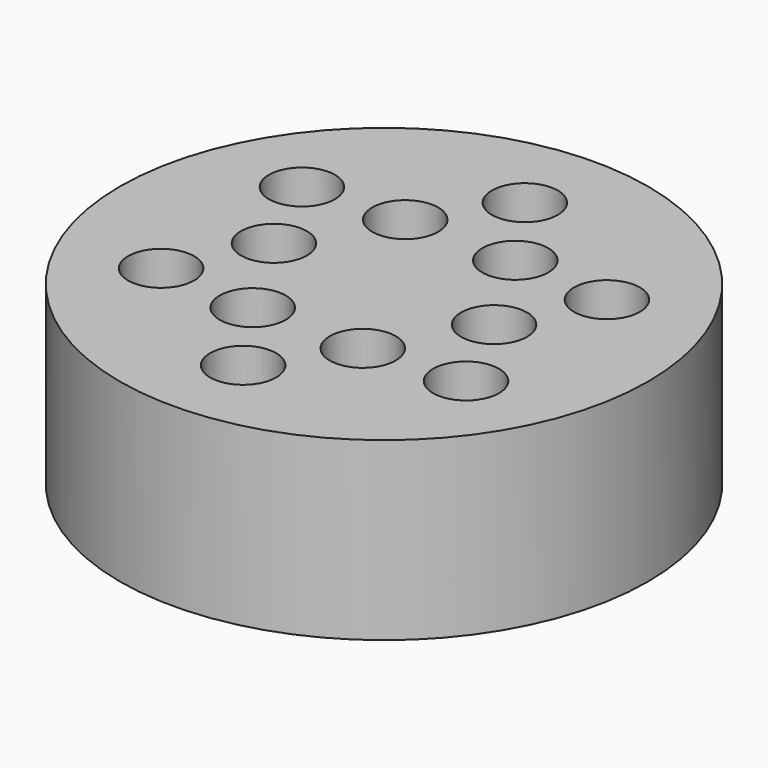
from build123d import *

# Parameters (mm, degrees)
F0_R     = 60
F1_DEPTH = 40
F2_R     = 7.5
F3_DEPTH = 25
F4_R     = 7.5
F5_DEPTH = 40.001


# Not quite as in the source:
# - a feature names something its author has since deleted; it is built from what else it names


with BuildPart() as f1:
    # F0 (on Top) → F1 (new body)
    with BuildSketch(Plane.XY):
        Circle(F0_R)
    extrude(amount=F1_DEPTH)

    # F2 (on face) → F3 (cut)
    with BuildSketch(Plane.XY.offset(40)):
        with Locations((-34.6410161514, 20)):
            Circle(F2_R)
        with Locations((0, 40)):
            Circle(F2_R)
        with Locations((34.6410161514, 20)):
            Circle(F2_R)
        with Locations((34.6410161514, -20)):
            Circle(F2_R)
        with Locations((0, -40)):
            Circle(F2_R)
        with Locations((-34.6410161514, -20)):
            Circle(F2_R)
    extrude(amount=-F3_DEPTH, mode=Mode.SUBTRACT)

    # F4 (on face) → F5 (cut, through all)
    with BuildSketch(Plane.XY.offset(40)):
        with Locations((-25, 0)):
            Circle(F4_R)
        with Locations((-12.5, -21.6506350946)):
            Circle(F4_R)
        with Locations((12.5, -21.6506350946)):
            Circle(F4_R)
        with Locations((25, 0)):
            Circle(F4_R)
        with Locations((12.5, 21.6506350946)):
            Circle(F4_R)
        with BuildLine():
            ThreePointArc((-8.75, 15.1554445662), (-6.0048094716, 17.9006350946), (-5, 21.6506350946))
            ThreePointArc((-5, 21.6506350946), (-18.9951905284, 25.4006350946), (-8.75, 15.1554445662))
        make_face()
    extrude(amount=-F5_DEPTH, mode=Mode.SUBTRACT)


solid = f1.part
